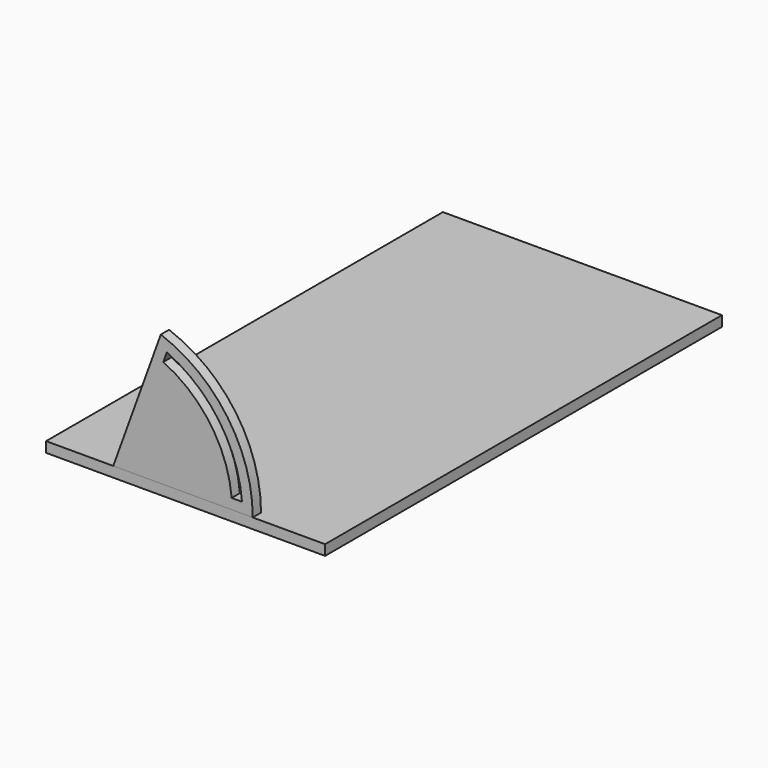
from build123d import *

# Parameters (mm, degrees)
F2_DEPTH = 6.35
F3_DEPTH = 304.8


# Not quite as in the source:
# - a feature names something its author has since deleted; it is built from what else it names


with BuildPart() as f2:
    # F0 (on Front) → F2 (new body)
    with BuildSketch(Plane.XZ):
        with BuildLine():
            Line((39.1451127164, -22.7806820739), (45.4951127164, -22.7806820739))
            ThreePointArc((45.4951127164, -22.7806820739), (29.9606120641, 26.4338424724), (-11.012777078, 57.8117251134))
            Line((-11.012777078, 57.8117251134), (-13.1770074636, 51.8419171736))
            ThreePointArc((-13.1770074636, 51.8419171736), (-10.2137544615, 50.700080003), (-7.2985464975, 49.4406265478))
            ThreePointArc((-7.2985464975, 49.4406265478), (24.7598523038, 22.7904093477), (38.8907050107, -16.4306820739))
            ThreePointArc((38.8907050107, -16.4306820739), (39.0814852879, -19.603134935), (39.1451127164, -22.7806820739))
        make_face()
        with BuildLine():
            Line((-13.1770074636, 51.8419171736), (-15.3412378492, 45.8721092338))
            ThreePointArc((-15.3412378492, 45.8721092338), (-12.380476471, 44.7253246395), (-9.472363604, 43.4509218784))
            Line((-9.472363604, 43.4509218784), (-8.3852980682, 46.4462067606))
            Line((-8.3852980682, 46.4462067606), (-7.2985464975, 49.4406265478))
            ThreePointArc((-7.2985464975, 49.4406265478), (-10.2137544615, 50.700080003), (-13.1770074636, 51.8419171736))
        make_face()
        with BuildLine():
            Line((-15.3412378492, 45.8721092338), (-40.2298872836, -22.7806820739))
            Line((-40.2298872836, -22.7806820739), (-11.6548872836, -22.7806820739))
            Line((-11.6548872836, -22.7806820739), (32.7951127164, -22.7806820739))
            ThreePointArc((32.7951127164, -22.7806820739), (32.7259272318, -19.6026711567), (32.5185018738, -16.4306820739))
            ThreePointArc((32.5185018738, -16.4306820739), (19.5599121895, 19.1458072135), (-9.472363604, 43.4509218784))
            ThreePointArc((-9.472363604, 43.4509218784), (-12.380476471, 44.7253246395), (-15.3412378492, 45.8721092338))
        make_face()
        with BuildLine():
            Line((35.9701127164, -22.7806820739), (39.1451127164, -22.7806820739))
            ThreePointArc((39.1451127164, -22.7806820739), (39.0814852879, -19.603134935), (38.8907050107, -16.4306820739))
            Line((38.8907050107, -16.4306820739), (35.7050684351, -16.4306820739))
            Line((35.7050684351, -16.4306820739), (35.7046034422, -16.4306820739))
            Line((35.7046034422, -16.4306820739), (32.5185018738, -16.4306820739))
            ThreePointArc((32.5185018738, -16.4306820739), (32.7259272318, -19.6026711567), (32.7951127164, -22.7806820739))
            Line((32.7951127164, -22.7806820739), (35.9701127164, -22.7806820739))
        make_face()
    extrude(amount=-F2_DEPTH)


with BuildPart() as f3:
    # F0 (on Front) → F3 (new body)
    with BuildSketch(Plane.XZ):
        Polygon((-81.5048872836, -22.7806820739), (-81.5048872836, -29.1306820739), (89.9451127164, -29.1306820739), (89.9451127164, -22.7806820739), (45.4951127164, -22.7806820739), (39.1451127164, -22.7806820739), (35.9701127164, -22.7806820739), (32.7951127164, -22.7806820739), (-11.6548872836, -22.7806820739), (-40.2298872836, -22.7806820739), align=None)
    extrude(amount=-F3_DEPTH)


solid = Compound([f2.part, f3.part])
